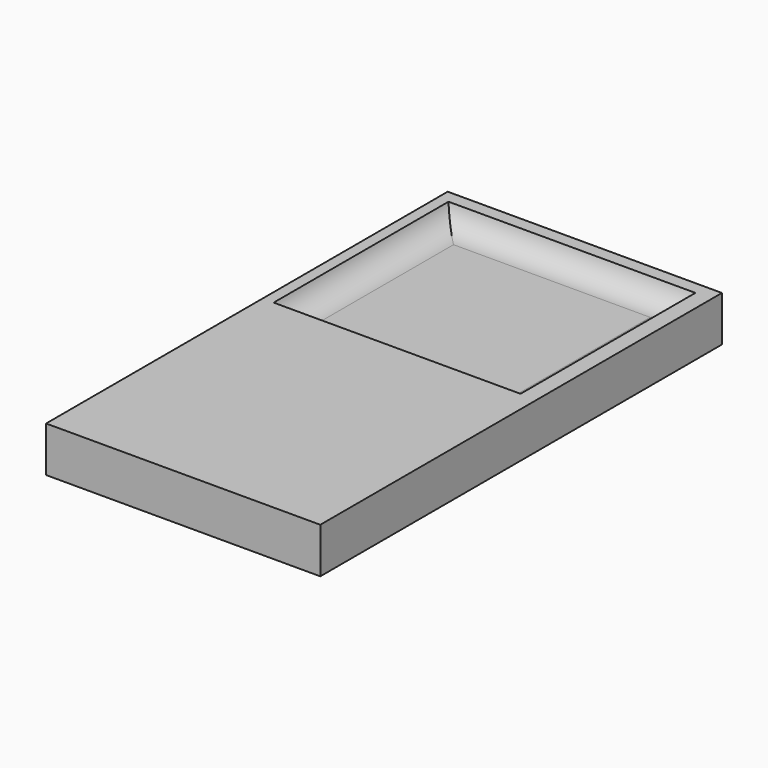
from build123d import *

# Parameters (mm, degrees)
F0_W        = 53.6803901196
F0_H        = 98.2824712992
F1_DEPTH    = 8.89
F2_W        = 48.3321249485
F2_H        = 42.7858147305
F3_DEPTH    = 3.81
F4_T1_DEPTH = 48.3321249485
F4_T3_DEPTH = 55.0825368547


# Not quite as in the source:
# - a fillet or chamfer that OpenCascade refuses, or shapes differently, is made with other operations: its cross-section is extruded or revolved along the edge and cut away or added


with BuildPart() as f1:
    # F0 (on Top) → F1 (new body)
    with BuildSketch(Plane.XY):
        Rectangle(F0_W, F0_H)
    extrude(amount=-F1_DEPTH)

    # F2 (on Top) → F3 (cut)
    with BuildSketch(Plane.XY):
        with Locations((-0.504437834, 25.230371044)):
            Rectangle(F2_W, F2_H)
    extrude(amount=-F3_DEPTH, mode=Mode.SUBTRACT)

    # F4: fillet of radius 5.08 on 4 edges, made by hand

    # F4_s2 → F4_t1 (join)
    with BuildSketch(Plane.YZ.offset(-24.6705003083)):
        with BuildLine():
            ThreePointArc((46.6232784092, 0), (44.8154415329, -2.7460926284), (41.7045895596, -3.81))
            Line((41.7045895596, -3.81), (46.6232784092, -3.81))
            Line((46.6232784092, -3.81), (46.6232784092, 0))
        make_face()
        with BuildLine():
            ThreePointArc((3.8374636788, 0), (5.6453005551, -2.7460926284), (8.7561525285, -3.81))
            Line((8.7561525285, -3.81), (3.8374636788, -3.81))
            Line((3.8374636788, -3.81), (3.8374636788, 0))
        make_face()
    extrude(amount=F4_T1_DEPTH)

    # F4_s4 → F4_t3 (join)
    with BuildSketch(Plane.XZ.offset(-46.6232784092)):
        with BuildLine():
            ThreePointArc((-24.6705003083, 0), (-22.8626634319, -2.7460926284), (-19.7518114586, -3.81))
            Line((-19.7518114586, -3.81), (-24.6705003083, -3.81))
            Line((-24.6705003083, -3.81), (-24.6705003083, 0))
        make_face()
        with BuildLine():
            ThreePointArc((23.6616246402, 0), (21.8537877639, -2.7460926284), (18.7429357905, -3.81))
            Line((18.7429357905, -3.81), (23.6616246402, -3.81))
            Line((23.6616246402, -3.81), (23.6616246402, 0))
        make_face()
    extrude(amount=F4_T3_DEPTH)


solid = f1.part
